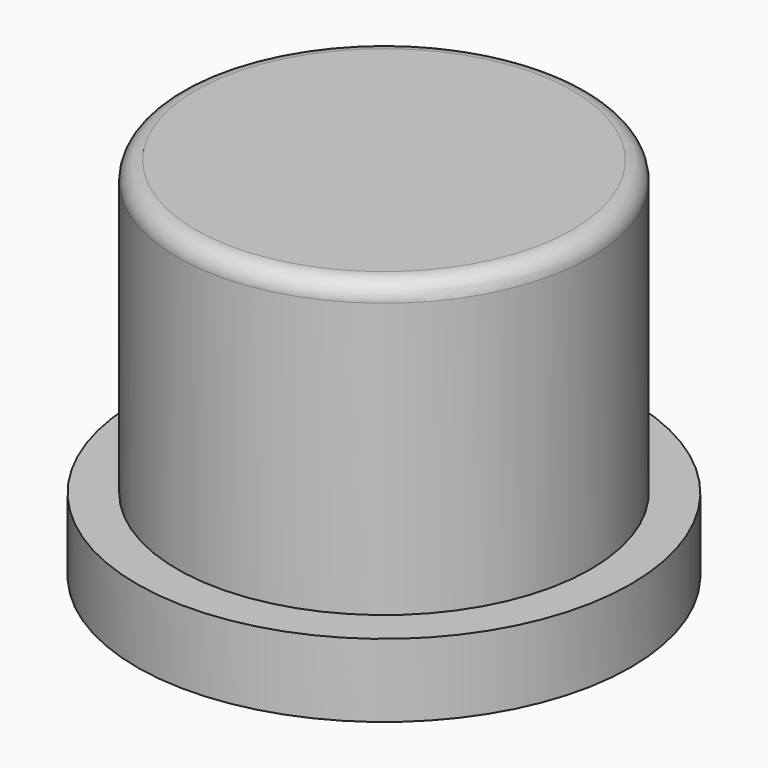
from build123d import *

# Parameters (mm, degrees)
F0_R         = 5.65
F0_TEXT_SIZE = 3.3189584584
F1_DEPTH     = 10
F0_R_2       = 6.75
F2_DEPTH     = 2
F3_R         = 0.5


# Not quite as in the source:
# - a feature names something its author has since deleted; it is built from what else it names
# - Text() gives the source's letters only with a copy of the font that has no kerning and outlines rounded to 1/6400 em; it was checked with that copy


with BuildPart() as f1:
    # F0 (on Top) → F1 (new body)
    with BuildSketch(Plane.XY):
        Circle(F0_R)
        with BuildLine():
            add(Edge.make_bspline(
                [(-2.80685354, 0.8385214331), (-2.4858480266, 0.5322956566), (-2.4858480266, -0.0174068381)],
                knots=[0, 0, 0, 1, 1, 1], degree=2))
            add(Edge.make_bspline(
                [(-2.4858480266, -0.0174068381), (-2.4858480266, -0.6023732664), (-2.8190403406, -0.9135256218)],
                knots=[0, 0, 0, 1, 1, 1], degree=2))
            add(Edge.make_bspline(
                [(-2.8190403406, -0.9135256218), (-3.1522326546, -1.2246779773), (-3.7807604127, -1.2246779773)],
                knots=[0, 0, 0, 1, 1, 1], degree=2))
            Line((-3.7807604127, -1.2246779773), (-4.451812326, -1.2246779773))
            Line((-4.451812326, -1.2246779773), (-4.451812326, 1.1447472096))
            Line((-4.451812326, 1.1447472096), (-3.7081581964, 1.1447472096))
            add(Edge.make_bspline(
                [(-3.7081581964, 1.1447472096), (-3.1278590534, 1.1447472096), (-2.80685354, 0.8385214331)],
                knots=[0, 0, 0, 1, 1, 1], degree=2))
        make_face(mode=Mode.SUBTRACT)
        with BuildLine():
            add(Edge.make_bspline(
                [(-0.4939543643, 0.1819899631), (-0.3871253889, -0.0303715195), (-0.3871253889, -0.3155945121)],
                knots=[0, 0, 0, 1, 1, 1], degree=2))
            add(Edge.make_bspline(
                [(-0.3871253889, -0.3155945121), (-0.3871253889, -0.7579494441), (-0.6204896555, -1.0076492094)],
                knots=[0, 0, 0, 1, 1, 1], degree=2))
            add(Edge.make_bspline(
                [(-0.6204896555, -1.0076492094), (-0.8538539222, -1.2573489746), (-1.2702794912, -1.2573489746)],
                knots=[0, 0, 0, 1, 1, 1], degree=2))
            add(Edge.make_bspline(
                [(-1.2702794912, -1.2573489746), (-1.5311288826, -1.2573489746), (-1.7305256837, -1.143000484)],
                knots=[0, 0, 0, 1, 1, 1], degree=2))
            add(Edge.make_bspline(
                [(-1.7305256837, -1.143000484), (-1.9299224849, -1.0286519934), (-2.0367514602, -0.814734749)],
                knots=[0, 0, 0, 1, 1, 1], degree=2))
            add(Edge.make_bspline(
                [(-2.0367514602, -0.814734749), (-2.1435804356, -0.6008175046), (-2.1435804356, -0.3155945121)],
                knots=[0, 0, 0, 1, 1, 1], degree=2))
            add(Edge.make_bspline(
                [(-2.1435804356, -0.3155945121), (-2.1435804356, 0.1283161817), (-1.9120312244, 0.3746451298)],
                knots=[0, 0, 0, 1, 1, 1], degree=2))
            add(Edge.make_bspline(
                [(-1.9120312244, 0.3746451298), (-1.6804820132, 0.6209740779), (-1.2604263333, 0.6209740779)],
                knots=[0, 0, 0, 1, 1, 1], degree=2))
            add(Edge.make_bspline(
                [(-1.2604263333, 0.6209740779), (-0.999576942, 0.6209740779), (-0.8001801408, 0.5076627618)],
                knots=[0, 0, 0, 1, 1, 1], degree=2))
            add(Edge.make_bspline(
                [(-0.8001801408, 0.5076627618), (-0.6007833397, 0.3943514457), (-0.4939543643, 0.1819899631)],
                knots=[0, 0, 0, 1, 1, 1], degree=2))
        make_face(mode=Mode.SUBTRACT)
        with BuildLine():
            Line((2.0486789672, -1.2246779773), (1.5109039795, -1.2246779773))
            Line((1.5109039795, -1.2246779773), (1.3714040068, -0.5909643467))
            Line((1.3714040068, -0.5909643467), (1.183675419, 0.2097343814))
            Line((1.183675419, 0.2097343814), (1.1722664993, 0.2097343814))
            Line((1.1722664993, 0.2097343814), (0.8414078279, -1.2246779773))
            Line((0.8414078279, -1.2246779773), (0.3098558873, -1.2246779773))
            Line((0.3098558873, -1.2246779773), (-0.205101261, 0.5872659061))
            Line((-0.205101261, 0.5872659061), (0.2875566352, 0.5872659061))
            Line((0.2875566352, 0.5872659061), (0.4965473006, -0.2149885838))
            add(Edge.make_bspline(
                [(0.4965473006, -0.2149885838), (0.5468502648, -0.4307208836), (0.5987089907, -0.80980817)],
                knots=[0, 0, 0, 1, 1, 1], degree=2))
            Line((0.5987089907, -0.80980817), (0.6080435613, -0.80980817))
            add(Edge.make_bspline(
                [(0.6080435613, -0.80980817), (0.6147851957, -0.6863844023), (0.6650881598, -0.4193119639)],
                knots=[0, 0, 0, 1, 1, 1], degree=2))
            Line((0.6650881598, -0.4193119639), (0.6910175228, -0.281367753))
            Line((0.6910175228, -0.281367753), (0.9145286315, 0.5872659061))
            Line((0.9145286315, 0.5872659061), (1.4590452536, 0.5872659061))
            Line((1.4590452536, 0.5872659061), (1.6711474425, -0.281367753))
            add(Edge.make_bspline(
                [(1.6711474425, -0.281367753), (1.6778890769, -0.3171502738), (1.6916316393, -0.3869002602)],
                knots=[0, 0, 0, 1, 1, 1], degree=2))
            add(Edge.make_bspline(
                [(1.6916316393, -0.3869002602), (1.7053742016, -0.4566502466), (1.7183388831, -0.5352162163)],
                knots=[0, 0, 0, 1, 1, 1], degree=2))
            add(Edge.make_bspline(
                [(1.7183388831, -0.5352162163), (1.7313035646, -0.6137821861), (1.7419346034, -0.6889773386)],
                knots=[0, 0, 0, 1, 1, 1], degree=2))
            add(Edge.make_bspline(
                [(1.7419346034, -0.6889773386), (1.7525656422, -0.7641724912), (1.754121404, -0.80980817)],
                knots=[0, 0, 0, 1, 1, 1], degree=2))
            Line((1.754121404, -0.80980817), (1.7634559747, -0.80980817))
            add(Edge.make_bspline(
                [(1.7634559747, -0.80980817), (1.7784950052, -0.6931260367), (1.8155739942, -0.4898398311)],
                knots=[0, 0, 0, 1, 1, 1], degree=2))
            add(Edge.make_bspline(
                [(1.8155739942, -0.4898398311), (1.8526529832, -0.2865536256), (1.8692477755, -0.2149885838)],
                knots=[0, 0, 0, 1, 1, 1], degree=2))
            Line((1.8692477755, -0.2149885838), (2.0860172498, 0.5872659061))
            Line((2.0860172498, 0.5872659061), (2.5708963371, 0.5872659061))
            Line((2.5708963371, 0.5872659061), (2.0486789672, -1.2246779773))
        make_face(mode=Mode.SUBTRACT)
        with BuildLine():
            Line((4.5347862875, -0.043336201), (4.5347862875, -1.2246779773))
            Line((4.5347862875, -1.2246779773), (4.0405726295, -1.2246779773))
            Line((4.0405726295, -1.2246779773), (4.0405726295, -0.1662413814))
            add(Edge.make_bspline(
                [(4.0405726295, -0.1662413814), (4.0405726295, 0.0297846025), (3.9708226432, 0.1277975945)],
                knots=[0, 0, 0, 1, 1, 1], degree=2))
            add(Edge.make_bspline(
                [(3.9708226432, 0.1277975945), (3.9010726568, 0.2258105865), (3.7486080026, 0.2258105865)],
                knots=[0, 0, 0, 1, 1, 1], degree=2))
            add(Edge.make_bspline(
                [(3.7486080026, 0.2258105865), (3.541173099, 0.2258105865), (3.4488645668, 0.0873477883)],
                knots=[0, 0, 0, 1, 1, 1], degree=2))
            add(Edge.make_bspline(
                [(3.4488645668, 0.0873477883), (3.3565560347, -0.0511150099), (3.3565560347, -0.3721205233)],
                knots=[0, 0, 0, 1, 1, 1], degree=2))
            Line((3.3565560347, -0.3721205233), (3.3565560347, -1.2246779773))
            Line((3.3565560347, -1.2246779773), (2.8623423768, -1.2246779773))
            Line((2.8623423768, -1.2246779773), (2.8623423768, 0.5872659061))
            Line((2.8623423768, 0.5872659061), (3.2398739014, 0.5872659061))
            Line((3.2398739014, 0.5872659061), (3.3062530706, 0.3554574012))
            Line((3.3062530706, 0.3554574012), (3.3337381953, 0.3554574012))
            add(Edge.make_bspline(
                [(3.3337381953, 0.3554574012), (3.4167121568, 0.4866599778), (3.5616572957, 0.5538170279)],
                knots=[0, 0, 0, 1, 1, 1], degree=2))
            add(Edge.make_bspline(
                [(3.5616572957, 0.5538170279), (3.7066024346, 0.6209740779), (3.8912194989, 0.6209740779)],
                knots=[0, 0, 0, 1, 1, 1], degree=2))
            add(Edge.make_bspline(
                [(3.8912194989, 0.6209740779), (4.207557727, 0.6209740779), (4.3711720072, 0.450099576)],
                knots=[0, 0, 0, 1, 1, 1], degree=2))
            add(Edge.make_bspline(
                [(4.3711720072, 0.450099576), (4.5347862875, 0.2792250742), (4.5347862875, -0.043336201)],
                knots=[0, 0, 0, 1, 1, 1], degree=2))
        make_face(mode=Mode.SUBTRACT)
        with BuildLine():
            add(Edge.make_bspline(
                [(-3.7340875594, -0.80980817), (-3.0080653966, -0.80980817), (-3.0080653966, -0.0303715195)],
                knots=[0, 0, 0, 1, 1, 1], degree=2))
            add(Edge.make_bspline(
                [(-3.0080653966, -0.0303715195), (-3.0080653966, 0.7329889259), (-3.6822288335, 0.7329889259)],
                knots=[0, 0, 0, 1, 1, 1], degree=2))
            Line((-3.6822288335, 0.7329889259), (-3.9493012719, 0.7329889259))
            Line((-3.9493012719, 0.7329889259), (-3.9493012719, -0.80980817))
            Line((-3.9493012719, -0.80980817), (-3.7340875594, -0.80980817))
        make_face()
        with BuildLine():
            add(Edge.make_bspline(
                [(-1.5523909602, 0.0889035501), (-1.640032207, -0.0448919628), (-1.640032207, -0.3155945121)],
                knots=[0, 0, 0, 1, 1, 1], degree=2))
            add(Edge.make_bspline(
                [(-1.640032207, -0.3155945121), (-1.640032207, -0.5847412996), (-1.5516130793, -0.7224262169)],
                knots=[0, 0, 0, 1, 1, 1], degree=2))
            add(Edge.make_bspline(
                [(-1.5516130793, -0.7224262169), (-1.4631939516, -0.8601111342), (-1.2640564441, -0.8601111342)],
                knots=[0, 0, 0, 1, 1, 1], degree=2))
            add(Edge.make_bspline(
                [(-1.2640564441, -0.8601111342), (-1.0659561111, -0.8601111342), (-0.9793520389, -0.7232040977)],
                knots=[0, 0, 0, 1, 1, 1], degree=2))
            add(Edge.make_bspline(
                [(-0.9793520389, -0.7232040977), (-0.8927479666, -0.5862970613), (-0.8927479666, -0.3155945121)],
                knots=[0, 0, 0, 1, 1, 1], degree=2))
            add(Edge.make_bspline(
                [(-0.8927479666, -0.3155945121), (-0.8927479666, -0.0464477246), (-0.9801299198, 0.0881256692)],
                knots=[0, 0, 0, 1, 1, 1], degree=2))
            add(Edge.make_bspline(
                [(-0.9801299198, 0.0881256692), (-1.0675118729, 0.2226990629), (-1.2671679677, 0.2226990629)],
                knots=[0, 0, 0, 1, 1, 1], degree=2))
            add(Edge.make_bspline(
                [(-1.2671679677, 0.2226990629), (-1.4647497134, 0.2226990629), (-1.5523909602, 0.0889035501)],
                knots=[0, 0, 0, 1, 1, 1], degree=2))
        make_face()
        with Locations((-4.75, -1.2246779773)):
            Text('Down', F0_TEXT_SIZE, font='Open Sans', font_style=FontStyle.BOLD, text_align=(TextAlign.LEFT, TextAlign.BOTTOM))
    extrude(amount=F1_DEPTH)

    # F0 (on Top) → F2 (join)
    with BuildSketch(Plane.XY):
        Circle(F0_R_2)
        Circle(F0_R, mode=Mode.SUBTRACT)
    extrude(amount=F2_DEPTH)

    # F3
    f3_edges = [f1.edges().sort_by_distance(p)[0] for p in [
        (-5.65, 0, 10),
    ]]
    fillet(f3_edges, radius=F3_R)


solid = f1.part
